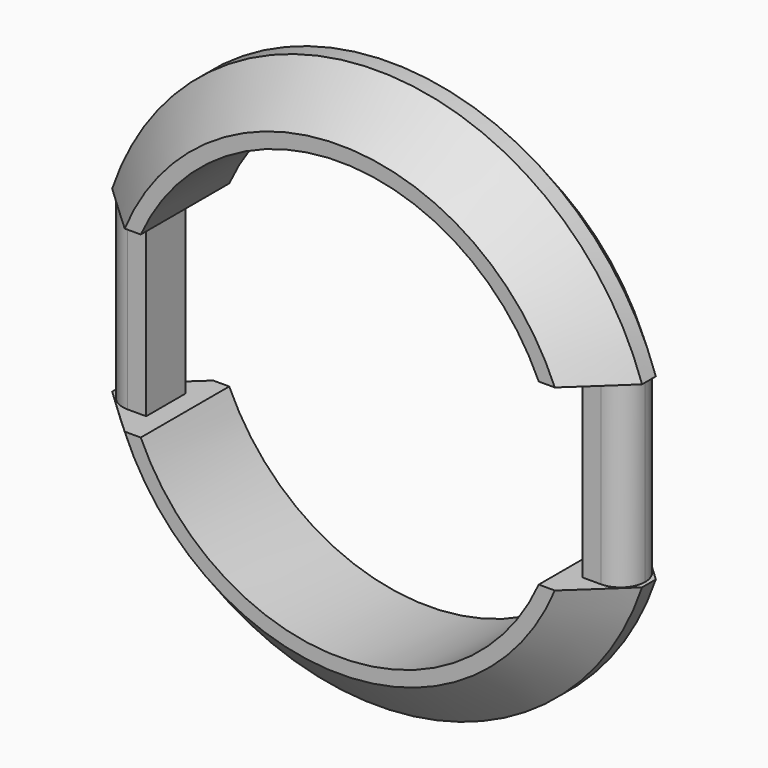
from build123d import *

# Parameters (mm, degrees)
F1_DEPTH      = 2.25
F1_DEPTH_BACK = 2.25
F2_DEPTH      = 1
F2_DEPTH_BACK = 1
F3_T2_ANGLE   = 191.9949180636
F3_T4_ANGLE   = 191.9949180636
F3_T6_ANGLE   = 191.9949180636
F3_T8_ANGLE   = 191.9949180636
F4_T4_DEPTH   = 11.4223278392
F4_T10_DEPTH  = 11.4223278392
F4_T16_DEPTH  = 11.4223278392
F4_T22_DEPTH  = 11.4223278392


# Not quite as in the source:
# - a fillet or chamfer that OpenCascade refuses, or shapes differently, is made with other operations: its cross-section is extruded or revolved along the edge and cut away or added


with BuildPart() as f1:
    # F0 (on Front) → F1 (new body, two sides)
    with BuildSketch(Plane.XZ) as f1_sk:
        with BuildLine():
            ThreePointArc((-8.0962065927, 3.6355279959), (0, 8.875), (8.0962065927, 3.6355279959))
            Line((8.0962065927, 3.6355279959), (8.875, 3.6355279959))
            Line((8.875, 3.6355279959), (10.625, 3.6355279959))
            Line((10.625, 3.6355279959), (10.7783839786, 3.6355279959))
            ThreePointArc((10.7783839786, 3.6355279959), (0, 11.375), (-10.7783839786, 3.6355279959))
            Line((-10.7783839786, 3.6355279959), (-10.625, 3.6355279959))
            Line((-10.625, 3.6355279959), (-8.875, 3.6355279959))
            Line((-8.875, 3.6355279959), (-8.0962065927, 3.6355279959))
        make_face()
    extrude(amount=F1_DEPTH)
    extrude(f1_sk.sketch, amount=-F1_DEPTH_BACK)



with BuildPart() as f1b:
    # F0 (on Front) → F1, piece 2 (new body, two sides)
    with BuildSketch(Plane.XZ) as f1_2_sk:
        with BuildLine():
            Line((8.875, -3.6355279959), (8.0962065927, -3.6355279959))
            ThreePointArc((8.0962065927, -3.6355279959), (0, -8.875), (-8.0962065927, -3.6355279959))
            Line((-8.0962065927, -3.6355279959), (-8.875, -3.6355279959))
            Line((-8.875, -3.6355279959), (-10.625, -3.6355279959))
            Line((-10.625, -3.6355279959), (-10.7783839786, -3.6355279959))
            ThreePointArc((-10.7783839786, -3.6355279959), (0, -11.375), (10.7783839786, -3.6355279959))
            Line((10.7783839786, -3.6355279959), (10.625, -3.6355279959))
            Line((10.625, -3.6355279959), (8.875, -3.6355279959))
        make_face()
    extrude(amount=F1_DEPTH)
    extrude(f1_2_sk.sketch, amount=-F1_DEPTH_BACK)


with BuildPart() as f1_1:
    add(f1.part)

    add(f1b.part)  # F2 merges F1b
    # F0 (on Front) → F2 (join, two sides)
    with BuildSketch(Plane.XZ) as f2_sk:
        Polygon((8.875, 3.6355279959), (8.875, 0), (8.875, -3.6355279959), (10.625, -3.6355279959), (10.625, 3.6355279959), align=None)
        Polygon((-8.875, -3.6355279959), (-8.875, 0), (-8.875, 3.6355279959), (-10.625, 3.6355279959), (-10.625, -3.6355279959), align=None)
    extrude(amount=F2_DEPTH)
    extrude(f2_sk.sketch, amount=-F2_DEPTH_BACK)

    # F3: chamfer of 1.9 on 4 edges, made by hand

    # F3_s1 → F3_t2 (revolve, cut)
    with BuildSketch(Plane(origin=(0, 0, 0), x_dir=(0, 1, 0), z_dir=(-0.1044843578, 0, -0.99452653))):
        Polygon((0.35, 11.375), (2.25, 9.475), (2.25, 11.375), align=None)
    revolve(axis=Axis((0, 2.25, 0), (0, -1, 0)), revolution_arc=F3_T2_ANGLE, mode=Mode.SUBTRACT)

    # F3_s3 → F3_t4 (revolve, cut)
    with BuildSketch(Plane(origin=(0, 0, 0), x_dir=(0, 1, 0), z_dir=(0.1044843578, 0, 0.99452653))):
        Polygon((2.25, 9.475), (0.35, 11.375), (2.25, 11.375), align=None)
    revolve(axis=Axis((0, 2.25, 0), (0, -1, 0)), revolution_arc=F3_T4_ANGLE, mode=Mode.SUBTRACT)

    # F3_s5 → F3_t6 (revolve, cut)
    with BuildSketch(Plane(origin=(0, 0, 0), x_dir=(0, 1, 0), z_dir=(-0.1044843578, 0, -0.99452653))):
        Polygon((-0.35, 11.375), (-2.25, 9.475), (-2.25, 11.375), align=None)
    revolve(axis=Axis((0, -2.25, 0), (0, -1, 0)), revolution_arc=F3_T6_ANGLE, mode=Mode.SUBTRACT)

    # F3_s7 → F3_t8 (revolve, cut)
    with BuildSketch(Plane(origin=(0, 0, 0), x_dir=(0, 1, 0), z_dir=(0.1044843578, 0, 0.99452653))):
        Polygon((-2.25, 9.475), (-0.35, 11.375), (-2.25, 11.375), align=None)
    revolve(axis=Axis((0, -2.25, 0), (0, -1, 0)), revolution_arc=F3_T8_ANGLE, mode=Mode.SUBTRACT)

    # F4: fillet of radius 1 on 4 edges, made by hand


with BuildPart() as f4_tool2:
    # F4_s3 → F4_t4 (new body)
    with BuildSketch(Plane.XY.offset(-5.7111639196)):
        with BuildLine():
            ThreePointArc((10.625, 0), (10.3321067812, -0.7071067812), (9.625, -1))
            Line((9.625, -1), (10.625, -1))
            Line((10.625, -1), (10.625, 0))
        make_face()
    extrude(amount=F4_T4_DEPTH)

    split(bisect_by=Plane.XY.offset(-3.6355279959), keep=Keep.TOP)

    split(bisect_by=Plane.XY.offset(3.6355279959), keep=Keep.BOTTOM)


with BuildPart() as f1_2:
    add(f1_1.part)

    # F4_t1: cut F4_tool2
    add(f4_tool2.part, mode=Mode.SUBTRACT)


with BuildPart() as f4_tool8:
    # F4_s9 → F4_t10 (new body)
    with BuildSketch(Plane.XY.offset(-5.7111639196)):
        with BuildLine():
            ThreePointArc((10.625, 0), (10.3321067812, 0.7071067812), (9.625, 1))
            Line((9.625, 1), (10.625, 1))
            Line((10.625, 1), (10.625, 0))
        make_face()
    extrude(amount=F4_T10_DEPTH)

    split(bisect_by=Plane.XY.offset(-3.6355279959), keep=Keep.TOP)

    split(bisect_by=Plane.XY.offset(3.6355279959), keep=Keep.BOTTOM)


with BuildPart() as f1_3:
    add(f1_2.part)

    # F4_t7: cut F4_tool8
    add(f4_tool8.part, mode=Mode.SUBTRACT)


with BuildPart() as f4_tool14:
    # F4_s15 → F4_t16 (new body)
    with BuildSketch(Plane.XY.offset(5.7111639196)):
        with BuildLine():
            ThreePointArc((-9.625, 1), (-10.3321067812, 0.7071067812), (-10.625, 0))
            Line((-10.625, 0), (-10.625, 1))
            Line((-10.625, 1), (-9.625, 1))
        make_face()
    extrude(amount=-F4_T16_DEPTH)

    split(bisect_by=Plane.XY.offset(-3.6355279959), keep=Keep.TOP)

    split(bisect_by=Plane.XY.offset(3.6355279959), keep=Keep.BOTTOM)


with BuildPart() as f1_4:
    add(f1_3.part)

    # F4_t13: cut F4_tool14
    add(f4_tool14.part, mode=Mode.SUBTRACT)


with BuildPart() as f4_tool20:
    # F4_s21 → F4_t22 (new body)
    with BuildSketch(Plane.XY.offset(5.7111639196)):
        with BuildLine():
            ThreePointArc((-9.625, -1), (-10.3321067812, -0.7071067812), (-10.625, 0))
            Line((-10.625, 0), (-10.625, -1))
            Line((-10.625, -1), (-9.625, -1))
        make_face()
    extrude(amount=-F4_T22_DEPTH)

    split(bisect_by=Plane.XY.offset(-3.6355279959), keep=Keep.TOP)

    split(bisect_by=Plane.XY.offset(3.6355279959), keep=Keep.BOTTOM)


with BuildPart() as f1_5:
    add(f1_4.part)

    # F4_t19: cut F4_tool20
    add(f4_tool20.part, mode=Mode.SUBTRACT)


solid = f1_5.part
